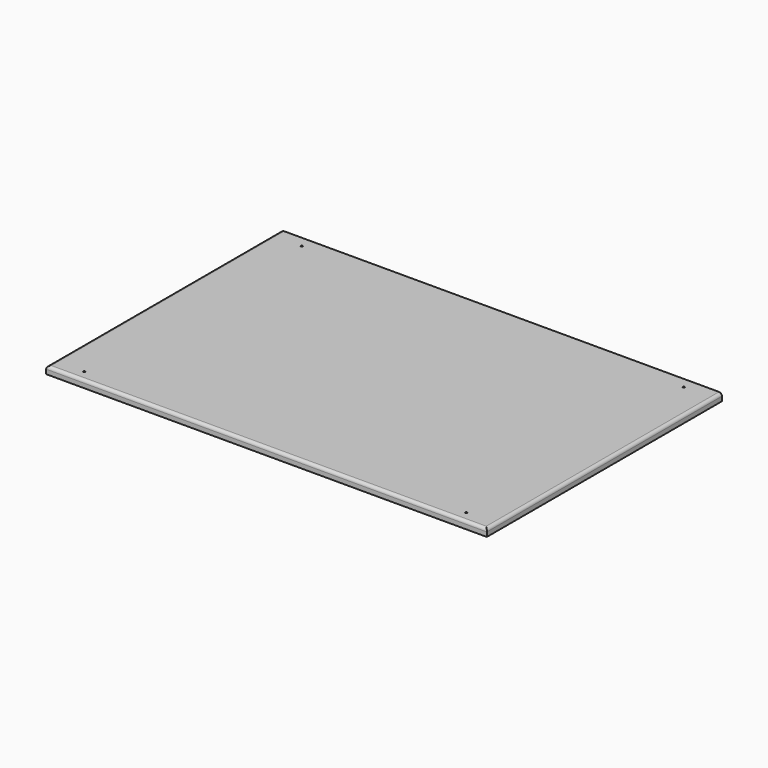
from build123d import *

# Parameters (mm, degrees)
F0_W      = 762
F0_H      = 508
F1_DEPTH  = 12.7
F2_R      = 5.08
F3_R      = 1.5875
F4_DEPTH  = 12.7
F5_R      = 1.5875
F6_DEPTH  = 12.7
F7_R      = 1.5875
F8_DEPTH  = 12.7
F9_R      = 1.5875
F10_DEPTH = 12.7


with BuildPart() as f1:
    # F0 (on Top) → F1 (new body)
    with BuildSketch(Plane.XY):
        Rectangle(F0_W, F0_H)
    extrude(amount=-F1_DEPTH)

    # F2
    f2_edges = [f1.edges().sort_by_distance(p)[0] for p in [
        (0, -254, 0),
        (381, 0, 0),
        (-381, 0, 0),
    ]]
    fillet(f2_edges, radius=F2_R)

    # F3 (on face) → F4 (cut, through all)
    with BuildSketch(Plane(origin=(0, 0, -12.7), x_dir=(1, 0, 0), z_dir=(0, 0, -1))):
        with Locations((330.2, 234.95)):
            Circle(F3_R)
    extrude(amount=-F4_DEPTH, mode=Mode.SUBTRACT)

    # F5 (on face) → F6 (cut, through all)
    with BuildSketch(Plane(origin=(0, 0, -12.7), x_dir=(1, 0, 0), z_dir=(0, 0, -1))):
        with Locations((-330.2, 234.95)):
            Circle(F5_R)
    extrude(amount=-F6_DEPTH, mode=Mode.SUBTRACT)

    # F7 (on face) → F8 (cut, through all)
    with BuildSketch(Plane(origin=(0, 0, -12.7), x_dir=(1, 0, 0), z_dir=(0, 0, -1))):
        with Locations((330.2, -234.95)):
            Circle(F7_R)
    extrude(amount=-F8_DEPTH, mode=Mode.SUBTRACT)

    # F9 (on face) → F10 (cut, through all)
    with BuildSketch(Plane(origin=(0, 0, -12.7), x_dir=(1, 0, 0), z_dir=(0, 0, -1))):
        with Locations((-330.2, -234.95)):
            Circle(F9_R)
    extrude(amount=-F10_DEPTH, mode=Mode.SUBTRACT)


solid = f1.part
